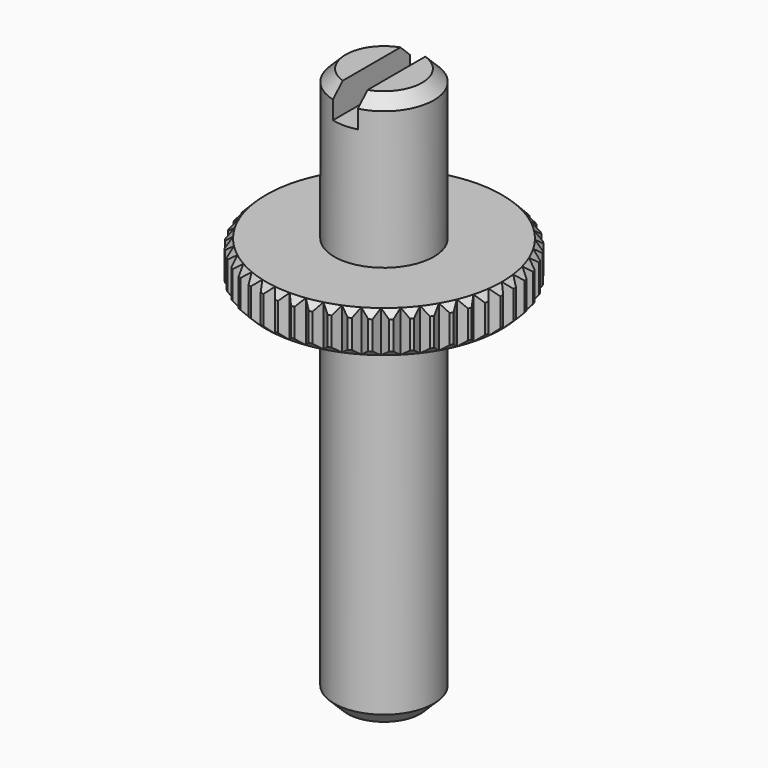
from build123d import *
from build123d import SkipClean  # not in build123d's __all__

# Parameters (mm, degrees)
F2_SIZE         = 0.8
F3_SIZE         = 0.7
F4_SIZE         = 0.4
F5_W            = 1.5
F5_H            = 1.8
F6_DEPTH        = 7.501
F6_DEPTH_BACK   = 7.501
F8_DEPTH        = 24.501
F8_COPIES_COUNT = 48


# Not quite as in the source:
# - a pattern or mirror of a feature is missing from the dataset's text; its kind, count and spacing are read off the source's solid


with BuildPart() as f1:
    # F0 (on Front) → F1 (revolve)
    with BuildSketch(Plane.XZ):
        Polygon((3, 9), (0, 9), (0, -24.5), (3, -24.5), (3, -2.5), (7.5, -2.5), (7.5, 0), (3, 0), align=None)
    revolve(axis=Axis((0, 0, 13.3836644055), (0, 0, 1)))

    # F2
    f2_edges = [f1.edges().sort_by_distance(p)[0] for p in [
        (-3, 0, -24.5),
    ]]
    chamfer(f2_edges, length=F2_SIZE)

    # F3
    f3_edges = [f1.edges().sort_by_distance(p)[0] for p in [
        (-3, 0, 9),
    ]]
    chamfer(f3_edges, length=F3_SIZE)

    # F4
    f4_edges = [f1.edges().sort_by_distance(p)[0] for p in [
        (-7.5, 0, -2.5),
        (-7.5, 0, 0),
    ]]
    chamfer(f4_edges, length=F4_SIZE)

    # F5 (on Front) → F6 (cut, two sides)
    with BuildSketch(Plane.XZ) as f6_sk:
        with Locations((0, 8.1)):
            Rectangle(F5_W, F5_H)
    extrude(amount=-F6_DEPTH, mode=Mode.SUBTRACT)
    extrude(f6_sk.sketch, amount=F6_DEPTH_BACK, mode=Mode.SUBTRACT)

    # F7 (on face) → F8 (cut, through all)
    with BuildSketch(Plane.XY):
        with BuildLine():
            Line((-0.3898604036, 7.4898604036), (0, 7.1))
            Line((0, 7.1), (0.3898604036, 7.4898604036))
            ThreePointArc((0.3898604036, 7.4898604036), (0, 7.5), (-0.3898604036, 7.4898604036))
        make_face()
    with SkipClean():  # cleaning this boolean's faces spoils the solid; the shape is the same uncleaned
        f8 = extrude(amount=-F8_DEPTH, mode=Mode.SUBTRACT)

    # F8_copies: F8 ×48 about axis
    f8_copies_axis = Axis((0, 0, 0), (0, 0, 1))
    for i in range(1, F8_COPIES_COUNT):
        add(f8.rotate(f8_copies_axis, i * 360 / F8_COPIES_COUNT), clean=False, mode=Mode.SUBTRACT)


solid = f1.part
